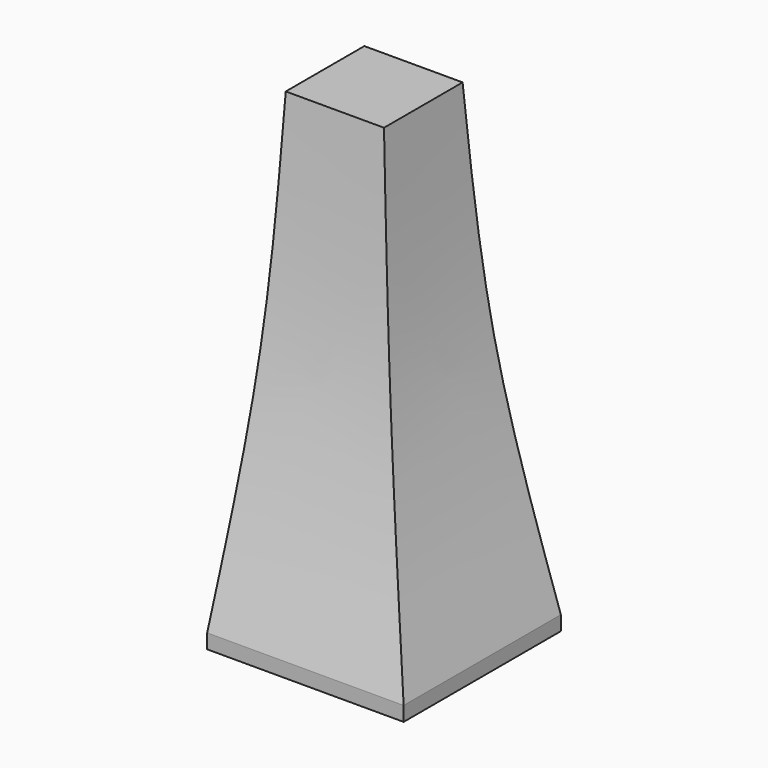
from build123d import *

# Parameters (mm, degrees)
F0_W     = 13.5
F0_H     = 13.5
F1_DEPTH = 30
F3_DEPTH = 13.5
F5_DEPTH = 13.5
F6_W     = 13.5
F6_H     = 13.5
F7_DEPTH = 1


# Not quite as in the source:
# - a feature names something its author has since deleted; it is built from what else it names


with BuildPart() as f1:
    # F0 (on Top) → F1 (new body)
    with BuildSketch(Plane.XY):
        with Locations((-6.75, 6.75)):
            Rectangle(F0_W, F0_H)
    extrude(amount=F1_DEPTH)

    # F2 (on face) → F3 (cut)
    with BuildSketch(Plane.XZ):
        with BuildLine():
            add(Edge.make_bspline(
                [(-6.75, 30), (-6.180103722, 24.9803399372), (-5.0311300437, 14.8601522679), (-1.6859534664, 4.9797013811), (0, 0)],
                knots=[0, 0, 0, 0, 0.4960046421, 1, 1, 1, 1], degree=3))
            Line((0, 0), (0, 30))
            Line((0, 30), (-6.75, 30))
        make_face()
    extrude(amount=-F3_DEPTH, mode=Mode.SUBTRACT)

    # F4 (on face) → F5 (cut)
    with BuildSketch(Plane(origin=(-13.5, 0, 0), x_dir=(0, -1, 0), z_dir=(-1, 0, 0))):
        with BuildLine():
            Line((0, 0), (0, 30))
            Line((0, 30), (-6.75, 30))
            add(Edge.make_bspline(
                [(-6.75, 30), (-6.180103722, 24.9803399372), (-5.0311300437, 14.8601522679), (-1.6859534664, 4.9797013811), (0, 0)],
                knots=[0, 0, 0, 0, 0.4960046421, 1, 1, 1, 1], degree=3))
        make_face()
    extrude(amount=-F5_DEPTH, mode=Mode.SUBTRACT)

    # F6 (on face) → F7 (join)
    with BuildSketch(Plane(origin=(0, 0, 0), x_dir=(1, 0, 0), z_dir=(0, 0, -1))):
        with Locations((-6.75, -6.75)):
            Rectangle(F6_W, F6_H)
    extrude(amount=F7_DEPTH)


solid = f1.part
